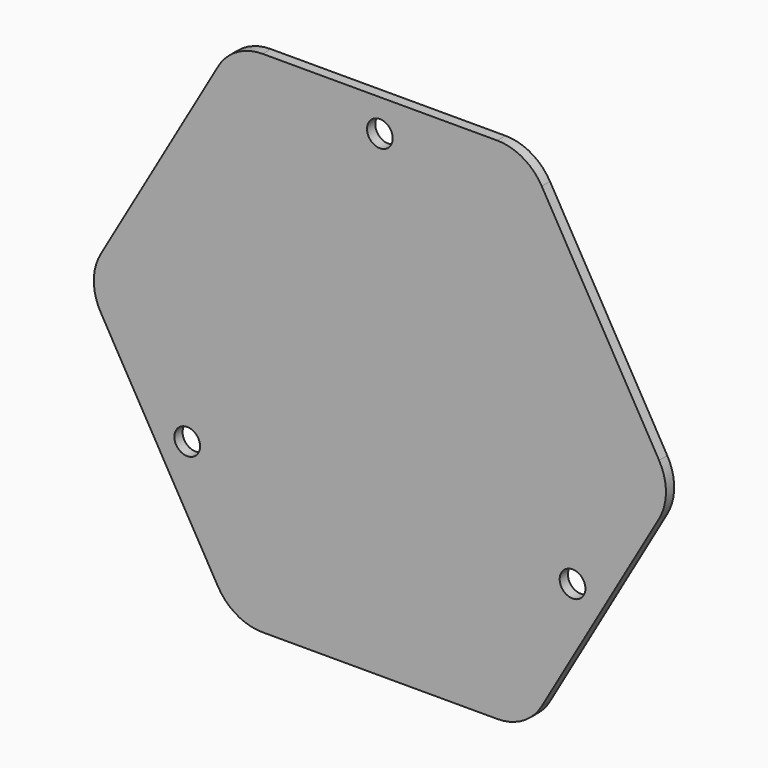
from build123d import *

# Parameters (mm, degrees)
F1_DEPTH = 5.08
F2_R     = 6.35
F3_DEPTH = 5.081


# Not quite as in the source:
# - a feature names something its author has since deleted; it is built from what else it names


with BuildPart() as f1:
    # F0 (on Front) → F1 (new body)
    with BuildSketch(Plane.XZ):
        with BuildLine():
            Line((137.8481502717, 12.7), (79.9225977639, 113.03))
            ThreePointArc((79.9225977639, 113.03), (70.6255525078, 122.3270452561), (57.9255525078, 125.73))
            Line((57.9255525078, 125.73), (-57.9255525078, 125.73))
            ThreePointArc((-57.9255525078, 125.73), (-70.6255525078, 122.3270452561), (-79.9225977639, 113.03))
            Line((-79.9225977639, 113.03), (-137.8481502717, 12.7))
            ThreePointArc((-137.8481502717, 12.7), (-141.2511050156, 0), (-137.8481502717, -12.7))
            Line((-137.8481502717, -12.7), (-79.9225977639, -113.03))
            ThreePointArc((-79.9225977639, -113.03), (-70.6255525078, -122.3270452561), (-57.9255525078, -125.73))
            Line((-57.9255525078, -125.73), (57.9255525078, -125.73))
            ThreePointArc((57.9255525078, -125.73), (70.6255525078, -122.3270452561), (79.9225977639, -113.03))
            Line((79.9225977639, -113.03), (137.8481502717, -12.7))
            ThreePointArc((137.8481502717, -12.7), (141.2511050156, 0), (137.8481502717, 12.7))
        make_face()
    extrude(amount=F1_DEPTH)

    # F2 (on face) → F3 (cut, through all)
    with BuildSketch(Plane.XZ.offset(5.08)):
        with Locations((0, 109.855)):
            Circle(F2_R)
        with Locations((-95.1372207327, -54.9275)):
            Circle(F2_R)
        with Locations((95.1372207327, -54.9275)):
            Circle(F2_R)
    extrude(amount=-F3_DEPTH, mode=Mode.SUBTRACT)


solid = f1.part
